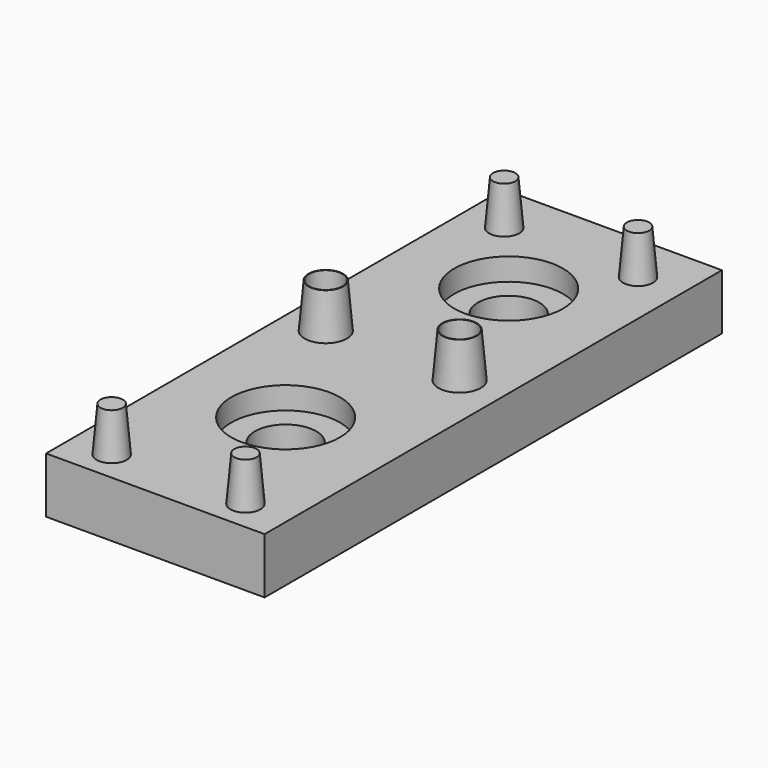
from build123d import *

# Parameters (mm, degrees)
F1_W           = 19.5961911231
F1_H           = 51.2615609914
F2_DEPTH       = 5
F3_R           = 1.35
F3_R_2         = 1.9
F4_DEPTH       = 4
F4_TAPER       = 5
F5_D           = 3
F5_DEPTH       = 25
F5_TIP         = 0.9012909285
F6_D           = 3.3
F6_DEPTH       = 25
F6_TIP         = 0.9914200214
F8_D           = 5.5
F8_DEPTH       = 25
F8_CBORE_D     = 9.75
F8_CBORE_DEPTH = 2
F8_TIP         = 1.6523667023


# Not quite as in the source:
# - a feature names something its author has since deleted; it is built from what else it names


with BuildPart() as f2:
    # F1 (on Top) → F2 (new body)
    with BuildSketch(Plane.XY):
        with Locations((0.1254314557, 10.8716255054)):
            Rectangle(F1_W, F1_H)
    extrude(amount=-F2_DEPTH)

    # F3 (on face) → F4 (join)
    with BuildSketch(Plane.XY):
        with Locations((-6, 32)):
            Circle(F3_R)
        with Locations((6, 32)):
            Circle(F3_R)
        with Locations((6, 12)):
            Circle(F3_R_2)
        with Locations((-6, 12)):
            Circle(F3_R_2)
        with Locations((6, -12)):
            Circle(F3_R)
        with Locations((-6, -12)):
            Circle(F3_R)
    extrude(amount=F4_DEPTH, taper=F4_TAPER)

    # F5 (one way)
    with BuildSketch(Plane(origin=(0, 0, 0), x_dir=(1, 0, 0), z_dir=(0, 0, -1))):
        with Locations((-6, -12), (6, -12)):
            Circle(F5_D / 2)
    extrude(amount=-F5_DEPTH, mode=Mode.SUBTRACT)
    with Locations(Plane(origin=(0, 0, 0), x_dir=(1, 0, 0), z_dir=(0, 0, -1))):
        with Locations((-6, -12), (6, -12)):
            with Locations((0, 0, -(F5_DEPTH + F5_TIP / 2))):  # 118° drill point
                Cone(0, F5_D / 2, F5_TIP, mode=Mode.SUBTRACT)

    # F6 (one way)
    with BuildSketch(Plane.XY):
        with Locations((6, 12), (-6, 12)):
            Circle(F6_D / 2)
    extrude(amount=-F6_DEPTH, mode=Mode.SUBTRACT)
    with Locations(Plane.XY):
        with Locations((6, 12), (-6, 12)):
            with Locations((0, 0, -(F6_DEPTH + F6_TIP / 2))):  # 118° drill point
                Cone(0, F6_D / 2, F6_TIP, mode=Mode.SUBTRACT)

    # F8
    with Locations(Plane.XY):
        with Locations((0, 0), (0, 25)):
            CounterBoreHole(F8_D / 2, F8_CBORE_D / 2, F8_CBORE_DEPTH, depth=F8_DEPTH)
            with Locations((0, 0, -(F8_DEPTH + F8_TIP / 2))):  # 118° drill point
                Cone(0, F8_D / 2, F8_TIP, mode=Mode.SUBTRACT)


solid = f2.part
